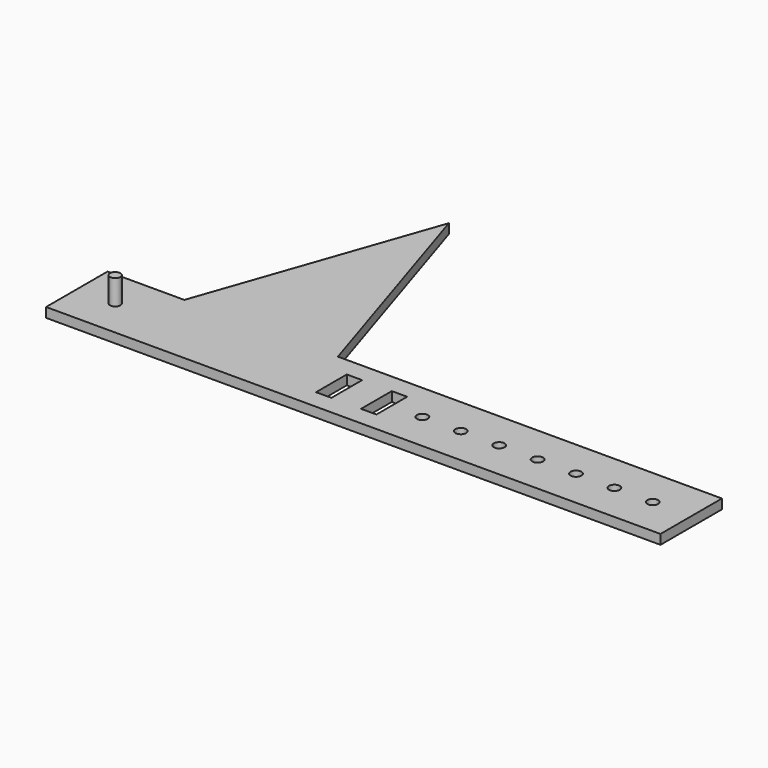
from build123d import *

# Parameters (mm, degrees)
F0_R     = 1.778
F0_W     = 19.05
F0_H     = 25.4
F0_R_2   = 1.7145
F1_DEPTH = 3.175
F2_DEPTH = 11.43


# Not quite as in the source:
# - a feature names something its author has since deleted; it is built from what else it names


with BuildPart() as f1:
    # F0 (on Top) → F1 (new body)
    with BuildSketch(Plane.XY):
        Polygon((-38.2503936946, 15.7646441165), (-38.2503936946, -9.6299967694), (139.5496063054, -9.6299967694), (139.5496063054, 15.7700032306), (12.5479004732, 15.7700032306), (-11.7069316009, 15.7700032306), (-38.2485270353, 15.7700032306), align=None)
        Polygon((20.5585099757, -3.2853558835), (20.5585099757, 3.0646441165), (20.5585099757, 9.4146441165), (25.6385099757, 9.4146441165), (25.6385099757, -3.2853558835), align=None, mode=Mode.SUBTRACT)
        Polygon((35.4481115937, -3.2853558835), (35.4481115937, 3.0646441165), (35.4481115937, 9.4146441165), (40.5281115937, 9.4146441165), (40.5281115937, -3.2853558835), align=None, mode=Mode.SUBTRACT)
        with Locations((50.6496063054, 3.0646441165)):
            Circle(F0_R, mode=Mode.SUBTRACT)
        with Locations((63.3496063054, 3.0646441165)):
            Circle(F0_R, mode=Mode.SUBTRACT)
        with Locations((76.0496063054, 3.0646441165)):
            Circle(F0_R, mode=Mode.SUBTRACT)
        with Locations((88.7496063054, 3.0646441165)):
            Circle(F0_R, mode=Mode.SUBTRACT)
        with Locations((101.4496063054, 3.0646441165)):
            Circle(F0_R, mode=Mode.SUBTRACT)
        with Locations((114.1496063054, 3.0646441165)):
            Circle(F0_R, mode=Mode.SUBTRACT)
        with Locations((126.8496063054, 3.0646441165)):
            Circle(F0_R, mode=Mode.SUBTRACT)
        Polygon((-44.6003936946, 15.7700032306), (-44.6003936946, -9.6299967694), (-38.2503936946, -9.6299967694), (-38.2503936946, 15.7646441165), (-38.2485270353, 15.7700032306), align=None)
        with Locations((-54.1253936946, 3.0700032306)):
            Rectangle(F0_W, F0_H)
        with Locations((-50.9503936946, 3.0646441165)):
            Circle(F0_R_2, mode=Mode.SUBTRACT)
        Polygon((-11.7069316009, 91.9700032306), (-38.2485270353, 15.7700032306), (-11.7069316009, 15.7700032306), align=None)
        Polygon((-11.7069316009, 91.9700032306), (-11.7069316009, 15.7700032306), (12.5479004732, 15.7700032306), align=None)
    extrude(amount=F1_DEPTH)

    # F0 (on Top) → F2 (join)
    with BuildSketch(Plane.XY):
        with Locations((-50.9503936946, 3.0646441165)):
            Circle(F0_R_2)
    extrude(amount=F2_DEPTH)


solid = f1.part
